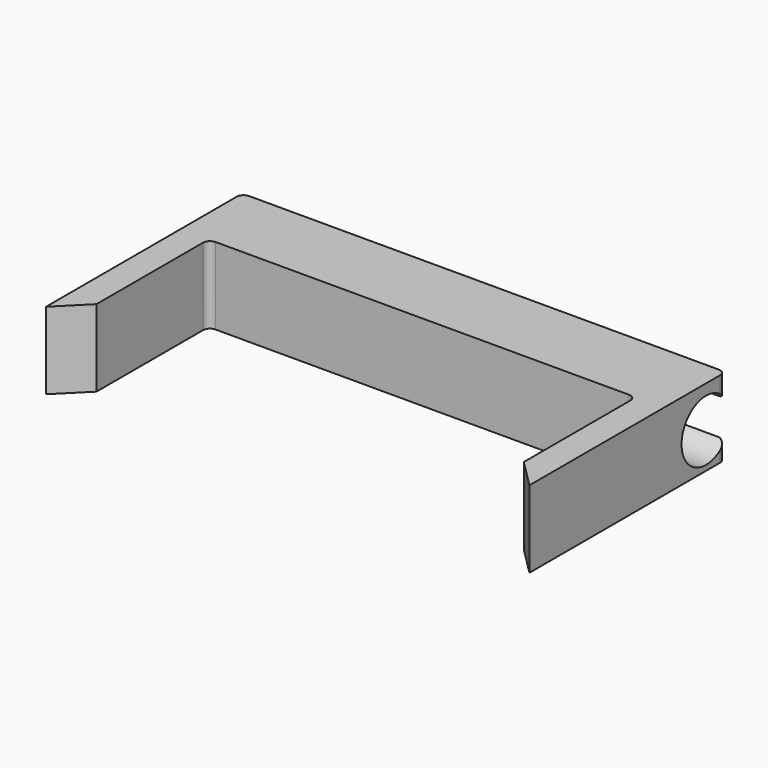
from build123d import *

# Parameters (mm, degrees)
F1_DEPTH    = 11
F2_T1_DEPTH = 36.7168298797
F3_R        = 4.35
F4_DEPTH    = 69.001
F5_T1_DEPTH = 36.7168298797
F6_R        = 1


# Not quite as in the source:
# - a fillet or chamfer that OpenCascade refuses, or shapes differently, is made with other operations: its cross-section is extruded or revolved along the edge and cut away or added


with BuildPart() as f1:
    # F0 (on Top) → F1 (new body)
    with BuildSketch(Plane.XY):
        Polygon((-65, -25), (-61, -25), (-61, 0), (0, 0), (0, -25), (4, -25), (4, 11), (-65, 11), align=None)
    extrude(amount=F1_DEPTH)

    # F2: chamfer of 5 on 1 edges, made by hand

    # F2_s2 → F2_t1 (cut)
    with BuildSketch(Plane.XY.offset(-12.8584149398)):
        Polygon((0, -20), (5, -25), (0, -25), align=None)
    extrude(amount=F2_T1_DEPTH, mode=Mode.SUBTRACT)

    # F3 (on face) → F4 (cut, through all)
    with BuildSketch(Plane(origin=(-65, 0, 0), x_dir=(0, -1, 0), z_dir=(-1, 0, 0))):
        with Locations((-7.5, 5.0990604796)):
            Circle(F3_R)
    extrude(amount=-F4_DEPTH, mode=Mode.SUBTRACT)

    # F5: chamfer of 5 on 1 edges, made by hand

    # F5_s2 → F5_t1 (cut)
    with BuildSketch(Plane.XY.offset(-12.8584149398)):
        Polygon((-66, -25), (-61, -20), (-61, -25), align=None)
    extrude(amount=F5_T1_DEPTH, mode=Mode.SUBTRACT)

    # F6
    f6_edges = [f1.edges().sort_by_distance(p)[0] for p in [
        (-61, 0, 5.5),
        (0, 0, 5.5),
        (4, 11, 9.341089),
        (4, 11, 1.257971),
        (-65, 11, 9.341089),
        (-65, 11, 1.257971),
    ]]
    fillet(f6_edges, radius=F6_R)


solid = f1.part
